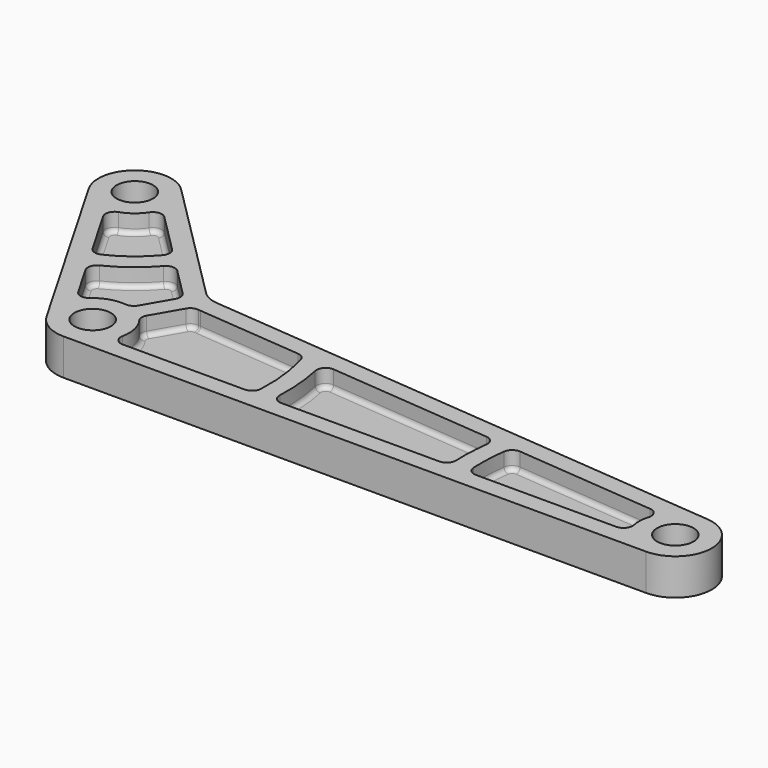
from build123d import *

# Parameters (mm, degrees)
F5_DEPTH   = 4
F6_DEPTH   = 2
F7_R       = 1
F8_D       = 4
F8_ON_F4_D = 4
F9_R       = 0.5


with BuildPart() as f5:
    # F3 (on Top) → F5 (new body)
    with BuildSketch(Plane.XY):
        with BuildLine():
            ThreePointArc((-9.1715728753, 23.6130368156), (-14.435045716, 23.958023052), (-15.4641016151, 18.7846096908))
            Line((-15.4641016151, 18.7846096908), (-3.4641016151, -2))
            ThreePointArc((-3.4641016151, -2), (-2, -3.4641016151), (0, -4))
            Line((0, -4), (64, -4))
            ThreePointArc((64, -4), (67.9961878605, -0.1745926209), (64.3488524562, 3.9847587084))
            Line((64.3488524562, 3.9847587084), (6.3735953844, 9.0603008696))
            ThreePointArc((6.3735953844, 9.0603008696), (5.3673016496, 9.3299830492), (4.513914383, 9.9275495573))
            Line((4.513914383, 9.9275495573), (-9.1715728753, 23.6130368156))
        make_face()
        with BuildLine():
            Line((-1.7320508076, -1), (-13.7320508076, 19.7846096908))
            ThreePointArc((-13.7320508076, 19.7846096908), (-13.217522858, 22.3713163714), (-10.5857864376, 22.1988232532))
            Line((-10.5857864376, 22.1988232532), (3.0997008206, 8.513335995))
            ThreePointArc((3.0997008206, 8.513335995), (4.5220129317, 7.5173918147), (6.1991691563, 7.0679215155))
            Line((6.1991691563, 7.0679215155), (64.1744262281, 1.9923793542))
            ThreePointArc((64.1744262281, 1.9923793542), (65.9980939303, -0.0872963105), (64, -2))
            Line((64, -2), (0, -2))
            ThreePointArc((0, -2), (-1, -1.7320508076), (-1.7320508076, -1))
        make_face(mode=Mode.SUBTRACT)
        with BuildLine():
            ThreePointArc((-10.5857864376, 22.1988232532), (-13.217522858, 22.3713163714), (-13.7320508076, 19.7846096908))
            Line((-13.7320508076, 19.7846096908), (-1.7320508076, -1))
            ThreePointArc((-1.7320508076, -1), (-1, -1.7320508076), (0, -2))
            Line((0, -2), (64, -2))
            ThreePointArc((64, -2), (65.9980939303, -0.0872963105), (64.1744262281, 1.9923793542))
            Line((64.1744262281, 1.9923793542), (6.1991691563, 7.0679215155))
            ThreePointArc((6.1991691563, 7.0679215155), (4.5220129317, 7.5173918147), (3.0997008206, 8.513335995))
            Line((3.0997008206, 8.513335995), (-10.5857864376, 22.1988232532))
        make_face()
    extrude(amount=-F5_DEPTH)

    # F4 (on Top) → F6 (cut)
    with BuildSketch(Plane.XY):
        with BuildLine():
            ThreePointArc((-10.7332285288, 16.9904971411), (-11.3515565531, 16.3965616309), (-11.2825610648, 15.5419690037))
            Line((-11.2825610648, 15.5419690037), (-7.8159710245, 9.5376589249))
            ThreePointArc((-7.8159710245, 9.5376589249), (-4.6948628519, 11.2643696073), (-2.2191861723, 13.8322229879))
            Line((-2.2191861723, 13.8322229879), (-7.1216848225, 18.7347216381))
            ThreePointArc((-7.1216848225, 18.7347216381), (-7.9293005657, 19.0225510099), (-8.6630332829, 18.5790138237))
            ThreePointArc((-8.6630332829, 18.5790138237), (-9.564954284, 17.6111963297), (-10.7332285288, 16.9904971411))
        make_face()
        with BuildLine():
            Line((59.2941134363, 2.4196346107), (43.0159786813, 3.8447315129))
            ThreePointArc((43.0159786813, 3.8447315129), (42.6869980771, 0.931160645), (42.7606235706, -2))
            Line((42.7606235706, -2), (59.1010205144, -2))
            ThreePointArc((59.1010205144, -2), (59.8756171837, -1.632455532), (60.0808164115, -0.8))
            ThreePointArc((60.0808164115, -0.8), (60.0038121395, 0.1745926209), (60.1655202578, 1.1387559469))
            ThreePointArc((60.1655202578, 1.1387559469), (60.0337039445, 1.9859356182), (59.2941134363, 2.4196346107))
        make_face()
        with BuildLine():
            ThreePointArc((-0.7878274665, 12.4008642821), (-3.4773399939, 9.6776629267), (-6.8038475773, 7.7846096908))
            Line((-6.8038475773, 7.7846096908), (-4.1815405504, 3.2426406871))
            ThreePointArc((-4.1815405504, 3.2426406871), (-3.4759393695, 2.7555925279), (-2.6524121173, 2.9941125497))
            ThreePointArc((-2.6524121173, 2.9941125497), (-1.2066556333, 3.8136573237), (0.4473896319, 3.9749015733))
            ThreePointArc((0.4473896319, 3.9749015733), (1.0099445985, 4.0759553043), (1.4252624437, 4.4686269666))
            Line((1.4252624437, 4.4686269666), (3.1362823061, 7.4322003011))
            ThreePointArc((3.1362823061, 7.4322003011), (3.2657432435, 8.0271052244), (3.0262052657, 8.5868315498))
            Line((3.0262052657, 8.5868315498), (-0.7878274665, 12.4008642821))
        make_face()
        with BuildLine():
            ThreePointArc((6.1991691563, 7.0679215155), (6.082717203, 7.0794912289), (5.9665679168, 7.0937831511))
            ThreePointArc((5.9665679168, 7.0937831511), (5.3919973762, 7.0003528899), (4.9668091511, 6.6027658012))
            Line((4.9668091511, 6.6027658012), (3.1573132513, 3.4686269666))
            ThreePointArc((3.1573132513, 3.4686269666), (3.024908539, 2.9126153308), (3.218670924, 2.3749015733))
            ThreePointArc((3.218670924, 2.3749015733), (3.9060519403, 0.8618342298), (3.9191835885, -0.8))
            ThreePointArc((3.9191835885, -0.8), (4.1243828163, -1.632455532), (4.8989794856, -2))
            Line((4.8989794856, -2), (19.2296068025, -2))
            ThreePointArc((19.2296068025, -2), (19.2248060192, 2.0456322501), (18.3781800681, 6.0016893591))
            Line((18.3781800681, 6.0016893591), (6.1991691563, 7.0679215155))
        make_face()
        with BuildLine():
            Line((41.0155455293, 4.0198628244), (20.525896406, 5.8136638914))
            ThreePointArc((20.525896406, 5.8136638914), (21.2449485668, 1.9399153345), (21.2393764294, -2))
            Line((21.2393764294, -2), (40.7525389678, -2))
            ThreePointArc((40.7525389678, -2), (40.6889041469, 1.0184569555), (41.0155455293, 4.0198628244))
        make_face()
    extrude(amount=-F6_DEPTH, mode=Mode.SUBTRACT)

    # F7
    f7_edges = [f5.edges().sort_by_distance(p)[0] for p in [
        (-6.803848, 7.78461, -1),
        (-0.787827, 12.400864, -1),
        (-7.815971, 9.537659, -1),
        (-2.219186, 13.832223, -1),
        (19.229607, -2, -1),
        (21.239376, -2, -1),
        (41.015546, 4.019863, -1),
        (40.752539, -2, -1),
        (43.015979, 3.844732, -1),
        (42.760624, -2, -1),
        (18.37818, 6.001689, -1),
        (20.525896, 5.813664, -1),
    ]]
    fillet(f7_edges, radius=F7_R)

    # F8 (through all)
    with Locations(Plane.XY):
        with Locations((-12, 20.7846096908), (0, 0)):
            Hole(F8_D / 2)

    # F8 on F4 (through all)
    with Locations(Plane.XY):
        with Locations((64, 0)):
            Hole(F8_ON_F4_D / 2)

    # F9
    f9_edges = [f5.edges().sort_by_distance(p)[0] for p in [
        (-9.768693, 12.919873, -2),
        (-7.691302, 9.844628, -2),
        (-11.351557, 16.396562, -2),
        (-4.694863, 11.26437, -2),
        (-9.564954, 17.611196, -2),
        (-2.547962, 13.791251, -2),
        (-7.929301, 19.022551, -2),
        (-4.980752, 16.593789, -2),
        (-3.47734, 9.677663, -2),
        (-0.74324, 11.908155, -2),
        (-6.339467, 7.614019, -2),
        (1.511712, 10.101325, -2),
        (-5.215138, 5.032884, -2),
        (3.265743, 8.027105, -2),
        (-3.475939, 2.755593, -2),
        (2.280772, 5.950414, -2),
        (-1.206656, 3.813657, -2),
        (1.009945, 4.075955, -2),
        (11.953194, 6.564176, -2),
        (18.255867, 5.836043, -2),
        (6.082717, 7.079491, -2),
        (19.210795, 2.173278, -2),
        (5.391997, 7.000353, -2),
        (18.993592, -1.726135, -2),
        (4.062061, 5.035696, -2),
        (11.60251, -2, -2),
        (3.024909, 2.912615, -2),
        (4.124383, -1.632456, -2),
        (3.906052, 0.861834, -2),
        (21.258982, 1.779548, -2),
        (21.084467, 5.357053, -2),
        (21.58817, -1.691095, -2),
        (30.937847, 4.902132, -2),
        (30.999079, -2, -2),
        (40.646205, 3.743446, -2),
        (40.408713, -1.692425, -2),
        (40.688904, 1.018457, -2),
        (51.618597, 3.091601, -2),
        (43.232162, 3.549037, -2),
        (60.033704, 1.985936, -2),
        (42.686998, 0.931161, -2),
        (60.003812, 0.174593, -2),
        (43.001772, -1.724286, -2),
        (59.875617, -1.632456, -2),
        (51.396146, -2, -2),
    ]]
    fillet(f9_edges, radius=F9_R)


solid = f5.part
